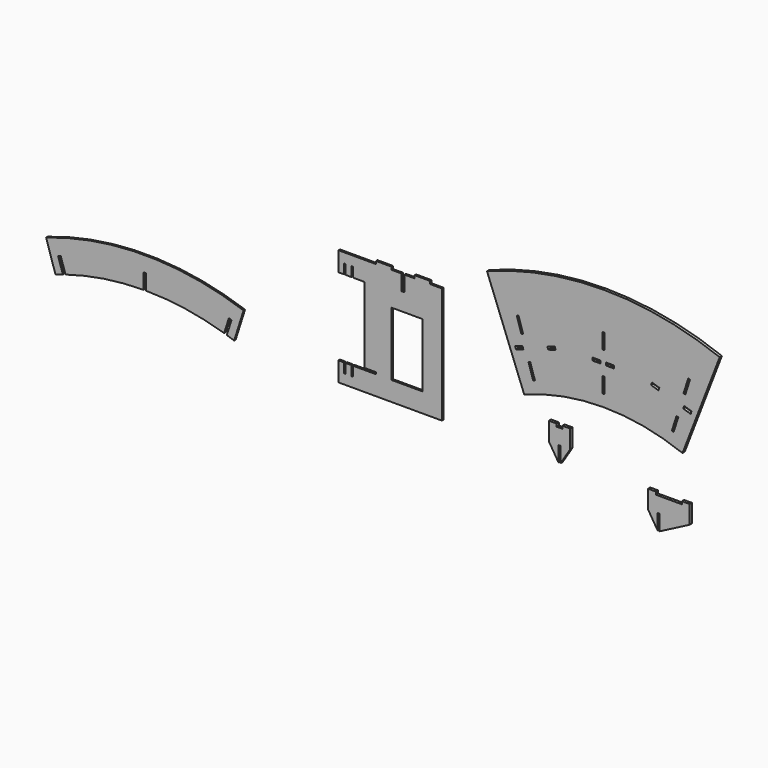
from build123d import *

# Parameters (mm, degrees)
F0_W     = 50.8
F0_H     = 18.1428571429
F1_DEPTH = 18.1356
F0_W_2   = 12.192
F0_H_2   = 101.6
F2_DEPTH = 12.192
F0_W_3   = 101.6


# Not quite as in the source:
# - a feature names something its author has since deleted; it is built from what else it names


with BuildPart() as f1:
    # F0 (on Front) → F1 (new body)
    with BuildSketch(Plane.XZ):
        Polygon((-245.2995117426, -748.2141169548), (-296.0995117426, -748.2141169548), (-296.0995117426, -849.8141169548), (-232.5995117426, -951.4141169548), (-232.5995117426, -849.8141169548), (-220.4075117426, -849.8141169548), (-220.4075117426, -951.4141169548), (-156.9075117426, -849.8141169548), (-156.9075117426, -748.2141169548), (-207.7075117426, -748.2141169548), align=None)
        with Locations((-182.3075117426, -739.1426883834)):
            Rectangle(F0_W, F0_H)
        with Locations((-270.6995117426, -739.1426883834)):
            Rectangle(F0_W, F0_H)
    extrude(amount=F1_DEPTH)


with BuildPart() as f1b:
    # F0 (on Front) → F1, piece 2 (new body)
    with BuildSketch(Plane.XZ):
        with BuildLine():
            Line((579.0676757709, -631.9954848741), (822.7111684876, 0))
            ThreePointArc((822.7111684876, 0), (60.7111684876, 141.7950471023), (-701.2888315124, 0))
            Line((-701.2888315124, 0), (-457.6453387957, -631.9954848741))
            ThreePointArc((-457.6453387957, -631.9954848741), (60.7111684876, -535.538286231), (579.0676757709, -631.9954848741))
        make_face()
        Polygon((-399.2400596646, -530.7352252686), (-430.0400842711, -433.9162266978), (-418.4218044426, -430.220223745), (-387.6217798361, -527.0392223158), align=None, mode=Mode.SUBTRACT)
        Polygon((-511.2292535926, -389.3006604553), (-516.7292579866, -372.0115535677), (-468.3197587013, -356.6115412645), (-462.8197543072, -373.9006481521), align=None, mode=Mode.SUBTRACT)
        Polygon((-464.6218413522, -284.9917258889), (-476.2401211807, -288.6877288417), (-507.0401457871, -191.8687302709), (-495.4218659586, -188.1727273182), align=None, mode=Mode.SUBTRACT)
        with Locations((60.7111684876, -408.5482073413)):
            Rectangle(F0_W_2, F0_H_2, mode=Mode.SUBTRACT)
        Polygon((539.8441414177, -430.220223745), (551.4624212462, -433.9162266978), (520.6623966398, -530.7352252686), (509.0441168113, -527.0392223158), align=None, mode=Mode.SUBTRACT)
        Polygon((589.7420956764, -356.6115412645), (638.1515949618, -372.0115535677), (632.6515905678, -389.3006604553), (584.2420912824, -373.9006481521), align=None, mode=Mode.SUBTRACT)
        Polygon((-300.3021495635, -322.2006068485), (-305.8021539575, -304.9114999608), (-257.3926546721, -289.5114876576), (-251.8926502781, -306.8005945453), align=None, mode=Mode.SUBTRACT)
        with Locations((16.5151684876, -281.5482073413)):
            Rectangle(F0_W, F0_H, mode=Mode.SUBTRACT)
        with Locations((104.9071684876, -281.5482073413)):
            Rectangle(F0_W, F0_H, mode=Mode.SUBTRACT)
        Polygon((373.3149872532, -306.8005945453), (378.8149916472, -289.5114876576), (427.2244909326, -304.9114999608), (421.7244865386, -322.2006068485), align=None, mode=Mode.SUBTRACT)
        Polygon((628.4624827623, -191.8687302709), (597.6624581558, -288.6877288417), (586.0441783273, -284.9917258889), (616.8442029338, -188.1727273182), align=None, mode=Mode.SUBTRACT)
        with Locations((60.7111684876, -154.5482073413)):
            Rectangle(F0_W_2, F0_H_2, mode=Mode.SUBTRACT)
    extrude(amount=F1_DEPTH)


with BuildPart() as f1c:
    # F0 (on Front) → F1, piece 3 (new body)
    with BuildSketch(Plane.XZ):
        with Locations((378.5851431642, -919.9377022879)):
            Rectangle(F0_W, F0_H)
        Polygon((403.9851431642, -929.0091308594), (353.1851431642, -929.0091308594), (353.1851431642, -1030.6091308594), (416.6851431642, -1132.2091308594), (416.6851431642, -1030.6091308594), (428.8771431642, -1030.6091308594), (428.8771431642, -1132.2091308594), (625.3280003071, -1030.6091308594), (625.3280003071, -929.0091308594), (574.5280003071, -929.0091308594), align=None)
        with Locations((599.9280003071, -919.9377022879)):
            Rectangle(F0_W, F0_H)
    extrude(amount=F1_DEPTH)


with BuildPart() as f2:
    # F0 (on Front) → F2 (new body)
    with BuildSketch(Plane.XZ):
        with BuildLine():
            Line((-2956.4141467797, -741.3827241583), (-2938.2712896368, -741.3827241583))
            Line((-2938.2712896368, -741.3827241583), (-2938.2712896368, -842.9827241583))
            Line((-2938.2712896368, -842.9827241583), (-2938.5207805782, -842.9827241583))
            ThreePointArc((-2938.5207805782, -842.9827241583), (-2680.2581818501, -863.2133164178), (-2427.7087045022, -920.8987414075))
            Line((-2427.7087045022, -920.8987414075), (-2427.6805354276, -920.8101927253))
            Line((-2427.6805354276, -920.8101927253), (-2396.8805108212, -823.9911941546))
            Line((-2396.8805108212, -823.9911941546), (-2379.5914039336, -829.4911985486))
            Line((-2379.5914039336, -829.4911985486), (-2410.39142854, -926.3101971193))
            ThreePointArc((-2410.39142854, -926.3101971193), (-2386.2394133775, -934.184590775), (-2362.202814439, -942.4045556973))
            Line((-2362.202814439, -942.4045556973), (-2361.9819292546, -941.7102094226))
            Line((-2361.9819292546, -941.7102094226), (-2331.1819046482, -844.8912108518))
            Line((-2331.1819046482, -844.8912108518), (-2300.5800248164, -748.6950747267))
            ThreePointArc((-2300.5800248164, -748.6950747267), (-2947.3427182083, -639.7607545087), (-3594.1054116001, -748.6950747267))
            Line((-3594.1054116001, -748.6950747267), (-3532.4826219776, -942.4045556973))
            ThreePointArc((-3532.4826219776, -942.4045556973), (-3508.446023039, -934.184590775), (-3484.2940078765, -926.3101971193))
            Line((-3484.2940078765, -926.3101971193), (-3515.0940324829, -829.4911985486))
            Line((-3515.0940324829, -829.4911985486), (-3497.8049255953, -823.9911941546))
            Line((-3497.8049255953, -823.9911941546), (-3467.0049009889, -920.8101927253))
            Line((-3467.0049009889, -920.8101927253), (-3466.9767319143, -920.8987414075))
            ThreePointArc((-3466.9767319143, -920.8987414075), (-3214.4272545664, -863.2133164178), (-2956.1646558383, -842.9827241583))
            Line((-2956.1646558383, -842.9827241583), (-2956.4141467797, -842.9827241583))
            Line((-2956.4141467797, -842.9827241583), (-2956.4141467797, -741.3827241583))
        make_face()
    extrude(amount=F2_DEPTH)


with BuildPart() as f2b:
    # F0 (on Front) → F2, piece 2 (new body)
    with BuildSketch(Plane.XZ):
        Polygon((-1433.7949680964, -199.4009857178), (-1509.9949680964, -199.4009857178), (-1679.3283014297, -199.4009857178), (-1679.3283014297, -326.4009857178), (-1641.2283014297, -326.4009857178), (-1641.2283014297, -262.9009857178), (-1632.3383014297, -262.9009857178), (-1632.3383014297, -326.4009857178), (-1594.2383014297, -326.4009857178), (-1594.2383014297, -262.9009857178), (-1585.3483014297, -262.9009857178), (-1585.3483014297, -326.4009857178), (-1509.9949680964, -326.4009857178), (-1509.9949680964, -822.2089857178), (-1433.7949680964, -822.2089857178), (-1433.7949680964, -834.4009857178), (-1509.9949680964, -834.4009857178), (-1585.3483014297, -834.4009857178), (-1585.3483014297, -897.9009857178), (-1594.2383014297, -897.9009857178), (-1594.2383014297, -834.4009857178), (-1632.3383014297, -834.4009857178), (-1632.3383014297, -897.9009857178), (-1641.2283014297, -897.9009857178), (-1641.2283014297, -834.4009857178), (-1679.3283014297, -834.4009857178), (-1679.3283014297, -961.4009857178), (-1509.9949680964, -961.4009857178), (-1001.9949680964, -961.4009857178), (-1001.9949680964, -199.4009857178), (-1078.1949680964, -199.4009857178), (-1179.7949680964, -199.4009857178), (-1246.923539525, -199.4009857178), (-1246.923539525, -301.0009857178), (-1265.0663966678, -301.0009857178), (-1265.0663966678, -199.4009857178), (-1332.1949680964, -199.4009857178), align=None)
        Polygon((-1332.1949680964, -815.8589857178), (-1332.1949680964, -417.1152714321), (-1128.9949680964, -417.1152714321), (-1128.9949680964, -834.4009857178), (-1332.1949680964, -834.4009857178), align=None, mode=Mode.SUBTRACT)
        with Locations((-1382.9949680964, -190.3295571463)):
            Rectangle(F0_W_3, F0_H)
        with Locations((-1128.9949680964, -190.3295571463)):
            Rectangle(F0_W_3, F0_H)
    extrude(amount=F2_DEPTH)


solid = Compound([f1.part, f1b.part, f1c.part, f2.part, f2b.part])
